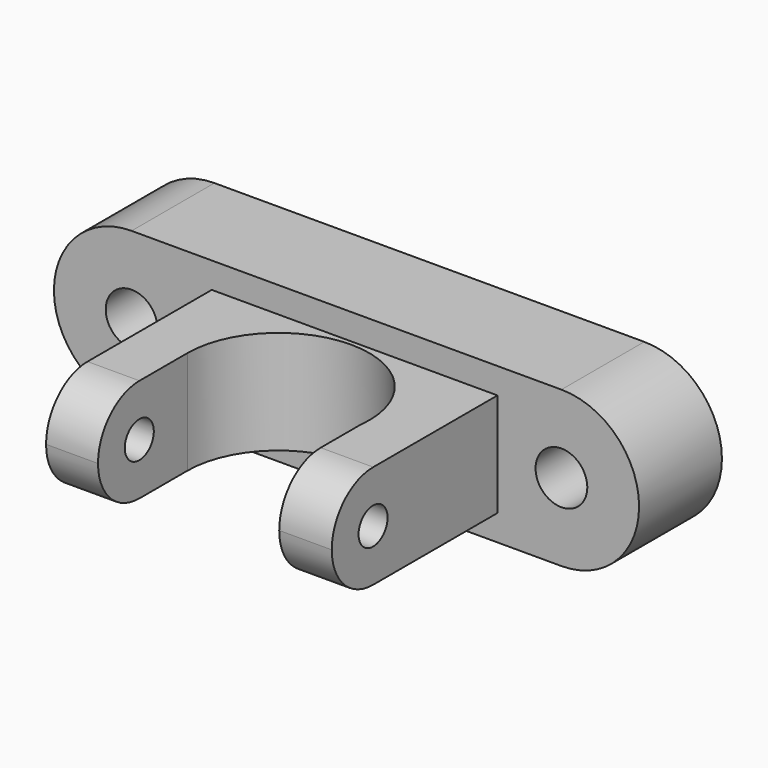
from build123d import *

# Parameters (mm, degrees)
F0_R     = 6.35
F1_DEPTH = 25.4
F2_W     = 70.0848072124
F2_H     = 25.4
F3_DEPTH = 50.8
F5_DEPTH = 25.4
F6_R     = 4.445
F7_DEPTH = 127
F8_R     = 12.69999


# Not quite as in the source:
# - a fillet or chamfer is up to 0.001 mm smaller than in the source, because OpenCascade refuses the exact size


with BuildPart() as f1:
    # F0 (on Front) → F1 (new body)
    with BuildSketch(Plane.XZ):
        with BuildLine():
            Line((-54.7069231111, -19.05), (50.7348023818, -19.05))
            ThreePointArc((50.7348023818, -19.05), (69.7848023818, 0), (50.7348023818, 19.05))
            Line((50.7348023818, 19.05), (-54.7069231111, 19.05))
            ThreePointArc((-54.7069231111, 19.05), (-73.7569231111, 0), (-54.7069231111, -19.05))
        make_face()
        with Locations((-54.7069231111, 0)):
            Circle(F0_R, mode=Mode.SUBTRACT)
        with Locations((50.7348023818, 0)):
            Circle(F0_R, mode=Mode.SUBTRACT)
    extrude(amount=F1_DEPTH)

    # F2 (on face) → F3 (join)
    with BuildSketch(Plane.XZ.offset(25.4)):
        Rectangle(F2_W, F2_H)
    extrude(amount=F3_DEPTH)

    # F4 (on face) → F5 (cut)
    with BuildSketch(Plane(origin=(0, 0, -12.7), x_dir=(1, 0, 0), z_dir=(0, 0, -1))):
        with BuildLine():
            Line((22.1503823996, 76.2), (-22.2996176004, 76.2))
            Line((-22.2996176004, 76.2), (-22.2996176004, 48.7618595362))
            ThreePointArc((-22.2996176004, 48.7618595362), (1.2899395164, 26.4995819984), (22.1503823996, 51.3374186365))
            Line((22.1503823996, 51.3374186365), (22.1503823996, 76.2))
        make_face()
    extrude(amount=-F5_DEPTH, mode=Mode.SUBTRACT)

    # F6 (on face) → F7 (cut)
    with BuildSketch(Plane(origin=(-35.0424036062, 0, 0), x_dir=(0, -1, 0), z_dir=(-1, 0, 0))):
        with Locations((63.5453920611, 0)):
            Circle(F6_R)
    extrude(amount=-F7_DEPTH, mode=Mode.SUBTRACT)

    # F8 (radius 12.7 in the source; OpenCascade refuses exactly that, so slightly less here)
    f8_edges = [f1.edges().sort_by_distance(p)[0] for p in [
        (-28.671011, -76.2, 12.7),
        (-28.671011, -76.2, -12.7),
        (28.596393, -76.2, 12.7),
        (28.596393, -76.2, -12.7),
    ]]
    fillet(f8_edges, radius=F8_R)


solid = f1.part
